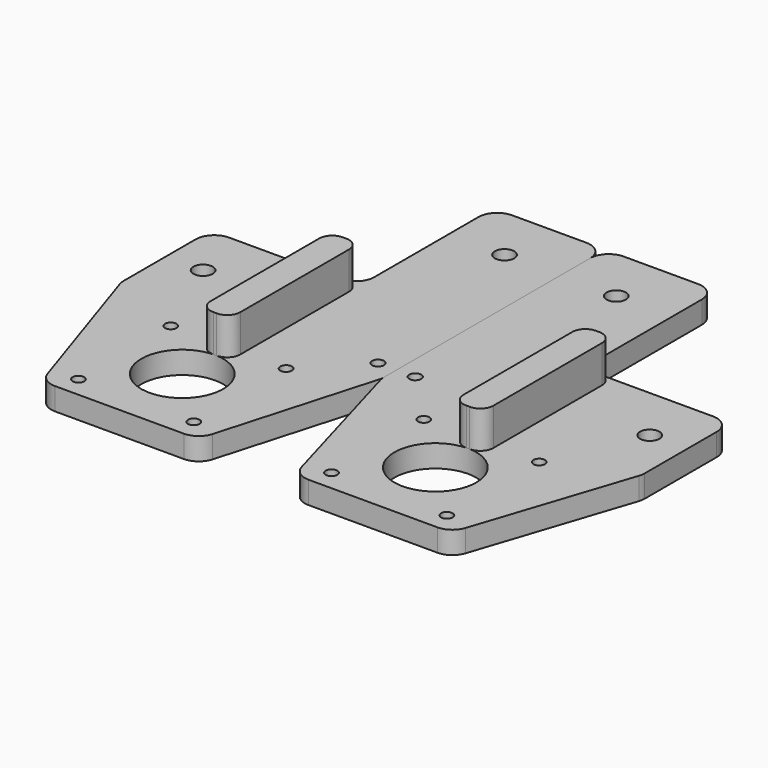
from build123d import *

# Parameters (mm, degrees)
F0_R        = 1.55
F0_R_2      = 11
F0_R_3      = 1.6
F0_R_4      = 2.6
F1_DEPTH    = 6
F3_DEPTH    = 10
F4_R        = 5
F5_T1_DEPTH = 18.75
F5_T3_DEPTH = 20.6110649506


# Not quite as in the source:
# - a fillet or chamfer that OpenCascade refuses, or shapes differently, is made with other operations: its cross-section is extruded or revolved along the edge and cut away or added


with BuildPart() as f1:
    # F0 (on Top) → F1 (new body)
    with BuildSketch(Plane.XY):
        Polygon((-22, -60.25), (20, -60.25), (35, -14.75), (35, 15.25), (-5, 15.25), (-5, 60.25), (-35, 60.25), (-35, -14.75), align=None)
        with Locations((-16.5, -54.75)):
            Circle(F0_R, mode=Mode.SUBTRACT)
        with Locations((-1, -39.25)):
            Circle(F0_R_2, mode=Mode.SUBTRACT)
        with Locations((-30, -9.75)):
            Circle(F0_R_3, mode=Mode.SUBTRACT)
        with Locations((-16.5, -23.75)):
            Circle(F0_R, mode=Mode.SUBTRACT)
        with Locations((14.5, -54.75)):
            Circle(F0_R, mode=Mode.SUBTRACT)
        with Locations((14.5, -23.75)):
            Circle(F0_R, mode=Mode.SUBTRACT)
        with Locations((-20, 45.25)):
            Circle(F0_R_4, mode=Mode.SUBTRACT)
        with Locations((25, 0.25)):
            Circle(F0_R_4, mode=Mode.SUBTRACT)
    extrude(amount=F1_DEPTH)

    # F2 (on face) → F3 (join)
    with BuildSketch(Plane.XY.offset(6)):
        with BuildLine():
            ThreePointArc((-5, -29.003049234), (-1, -28.25), (3, -29.003049234))
            Line((3, -29.003049234), (3, 15.25))
            Line((3, 15.25), (-5, 15.25))
            Line((-5, 15.25), (-5, -29.003049234))
        make_face()
    extrude(amount=F3_DEPTH)

    # F4
    f4_edges = [f1.edges().sort_by_distance(p)[0] for p in [
        (-35, 60.25, 3),
        (-5, 60.25, 3),
        (35, 15.25, 3),
        (-5, 15.25, 3),
        (20, -60.25, 3),
        (-22, -60.25, 3),
        (35, -14.75, 3),
        (-35, -14.75, 3),
    ]]
    fillet(f4_edges, radius=F4_R)

    # F5: fillet of radius 3.5 on 4 edges, made by hand

    # F5_s2 → F5_t1 (cut)
    with BuildSketch(Plane.XY.offset(6)):
        with BuildLine():
            ThreePointArc((-1.5, 15.25), (-3.9748737342, 14.2248737342), (-5, 11.75))
            Line((-5, 11.75), (-5, 15.25))
            Line((-5, 15.25), (-1.5, 15.25))
        make_face()
        with BuildLine():
            ThreePointArc((-0.5, 15.25), (1.9748737342, 14.2248737342), (3, 11.75))
            Line((3, 11.75), (3, 15.25))
            Line((3, 15.25), (-0.5, 15.25))
        make_face()
    extrude(amount=F5_T1_DEPTH, mode=Mode.SUBTRACT)

    # F5_s4 → F5_t3 (cut)
    with BuildSketch(Plane.XY.offset(6)):
        with BuildLine():
            ThreePointArc((-5, -24.7586232538), (-3.9318291682, -27.2758055866), (-1.3793103448, -28.2565417788))
            ThreePointArc((-1.3793103448, -28.2565417788), (-3.221240221, -28.4766025841), (-5, -29.003049234))
            Line((-5, -29.003049234), (-5, -24.7586232538))
        make_face()
        with BuildLine():
            ThreePointArc((3, -24.7586232538), (1.9318291682, -27.2758055866), (-0.6206896552, -28.2565417788))
            ThreePointArc((-0.6206896552, -28.2565417788), (1.221240221, -28.4766025841), (3, -29.003049234))
            Line((3, -29.003049234), (3, -24.7586232538))
        make_face()
    extrude(amount=F5_T3_DEPTH, mode=Mode.SUBTRACT)


with BuildPart() as f6_1:
    # F6: instance of F1
    add(f1.part.mirror(Plane(origin=(-35, 20.6001373616, 3), x_dir=(0, -1, 0), z_dir=(-1, 0, 0))))


solid = Compound([f1.part, f6_1.part])
